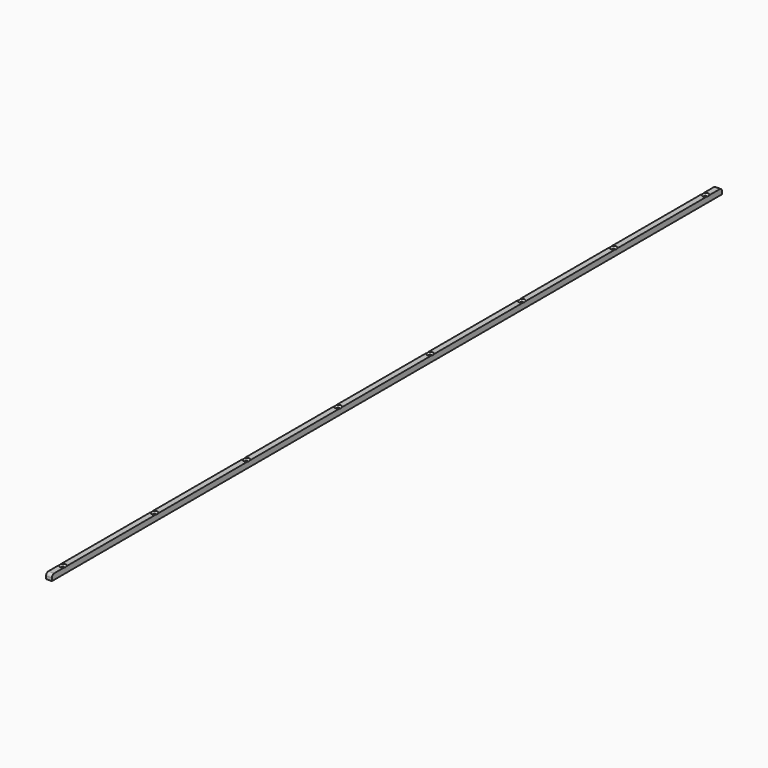
from build123d import *

# Parameters (mm, degrees)
F0_W           = 10
F0_H           = 10
F1_DEPTH       = 1460
F3_D           = 5.5
F3_CSINK_D     = 11.2
F3_CSINK_ANGLE = 90
F4_R           = 5
F5_R           = 5


# Not quite as in the source:
# - a feature names something its author has since deleted; it is built from what else it names


with BuildPart() as f1:
    # F0 (on Front) → F1 (new body)
    with BuildSketch(Plane.XZ):
        Rectangle(F0_W, F0_H)
    extrude(amount=-F1_DEPTH)

    # F3 (through all)
    with Locations(Plane.XY.offset(5)):
        with Locations((0, 30), (0, 230), (0, 430), (0, 630), (0, 830), (0, 1030), (0, 1230), (0, 1430)):
            CounterSinkHole(F3_D / 2, F3_CSINK_D / 2, counter_sink_angle=F3_CSINK_ANGLE)

    # F4
    f4_edges = [f1.edges().sort_by_distance(p)[0] for p in [
        (0, 1460, 5),
    ]]
    fillet(f4_edges, radius=F4_R)

    # F5
    f5_edges = [f1.edges().sort_by_distance(p)[0] for p in [
        (0, 0, 5),
    ]]
    fillet(f5_edges, radius=F5_R)


solid = f1.part
